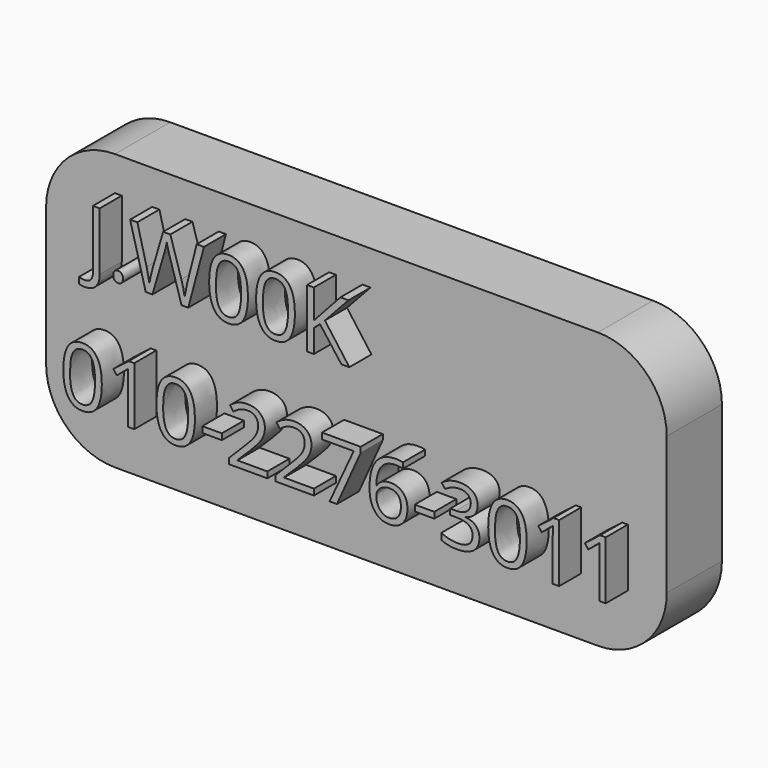
from build123d import *

# Parameters (mm, degrees)
F0_W         = 45
F0_H         = 20
F1_DEPTH     = 5
F2_R         = 5
F3_TEXT_SIZE = 5.9540422365
F4_DEPTH     = 2
F5_TEXT_SIZE = 5.90446756
F6_DEPTH     = 2


# Not quite as in the source:
# - Text() gives the source's letters only with a copy of the font that has no kerning and outlines rounded to 1/6400 em; it was checked with that copy


with BuildPart() as f1:
    # F0 (on Front) → F1 (new body)
    with BuildSketch(Plane.XZ):
        with Locations((22.5, 10)):
            Rectangle(F0_W, F0_H)
    extrude(amount=F1_DEPTH)

    # F2
    f2_edges = [f1.edges().sort_by_distance(p)[0] for p in [
        (45, -2.5, 20),
        (0, -2.5, 20),
        (45, -2.5, 0),
        (0, -2.5, 0),
    ]]
    fillet(f2_edges, radius=F2_R)

    # F3 (on face) → F4 (join)
    with BuildSketch(Plane.XZ.offset(5)):
        with Locations((4.4405241311, 13.2560484298)):
            Text('J.W00K', F3_TEXT_SIZE, font='Open Sans', text_align=(TextAlign.LEFT, TextAlign.BOTTOM))
    extrude(amount=F4_DEPTH)

    # F5 (on face) → F6 (join)
    with BuildSketch(Plane.XZ.offset(5)):
        with Locations((2.5573838579, 4.2264971173)):
            Text('010-2276-3011', F5_TEXT_SIZE, font='Open Sans', text_align=(TextAlign.LEFT, TextAlign.BOTTOM))
    extrude(amount=F6_DEPTH)


solid = f1.part
